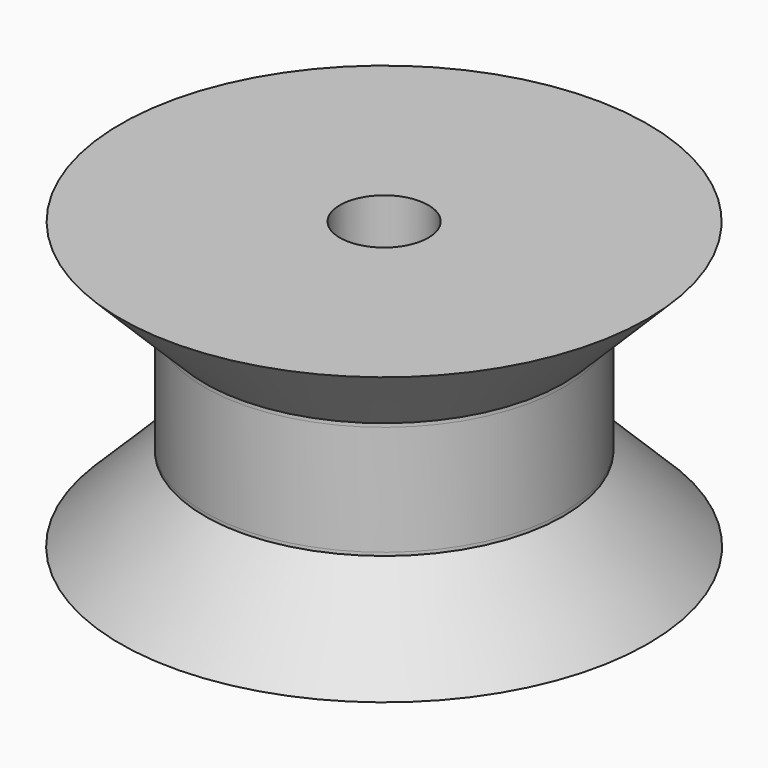
from build123d import *

# Parameters (mm, degrees)
F0_R        = 152.4
F1_DEPTH    = 50.8
F2_R        = 103.4812283395
F3_DEPTH    = 63.5
F5_R        = 152.1778472169
F6_DEPTH    = 50.8
F7_S5_R     = 103.4812283395
F7_T6_DEPTH = 218
F8_S5_R     = 103.4812283395
F8_T6_DEPTH = 219
F9_R        = 25.5370078958
F10_DEPTH   = 203.2


# Not quite as in the source:
# - a fillet or chamfer that OpenCascade refuses, or shapes differently, is made with other operations: its cross-section is extruded or revolved along the edge and cut away or added


with BuildPart() as f1:
    # F0 (on Top) → F1 (new body)
    with BuildSketch(Plane.XY):
        Circle(F0_R)
    extrude(amount=F1_DEPTH)

    # F2 (on face) → F3 (join)
    with BuildSketch(Plane.XY.offset(50.8)):
        Circle(F2_R)
    extrude(amount=F3_DEPTH)

    # F5 (on face) → F6 (join)
    with BuildSketch(Plane.XY.offset(114.3)):
        Circle(F5_R)
    extrude(amount=F6_DEPTH)

    # F7: chamfer of 50.8 on 1 edges, made by hand


with BuildPart() as f7_tool2:
    # F7_s3 → F7_t4 (revolve)
    with BuildSketch(Plane.XZ):
        Polygon((152.1778472169, 165.1), (101.3778472169, 114.3), (152.1778472169, 114.3), align=None)
    revolve(axis=Axis((0, 0, 114.3), (0, 0, 1)))

    # F7_s5 → F7_t6 (cut, symmetric)
    with BuildSketch(Plane.XY.offset(139.7)):
        Circle(F7_S5_R)
    extrude(amount=F7_T6_DEPTH, both=True, mode=Mode.SUBTRACT)


with BuildPart() as f1_1:
    add(f1.part)

    # F7_t1: cut F7_tool2
    add(f7_tool2.part, mode=Mode.SUBTRACT)

    # F8: chamfer of 50.8 on 1 edges, made by hand


with BuildPart() as f8_tool2:
    # F8_s3 → F8_t4 (revolve)
    with BuildSketch(Plane.XZ):
        Polygon((101.6, 50.8), (152.4, 0), (152.4, 50.8), align=None)
    revolve(axis=Axis((0, 0, 50.8), (0, 0, 1)))

    # F8_s5 → F8_t6 (cut, symmetric)
    with BuildSketch(Plane.XY.offset(25.4)):
        Circle(F8_S5_R)
    extrude(amount=F8_T6_DEPTH, both=True, mode=Mode.SUBTRACT)


with BuildPart() as f1_2:
    add(f1_1.part)

    # F8_t1: cut F8_tool2
    add(f8_tool2.part, mode=Mode.SUBTRACT)

    # F9 (on face) → F10 (cut)
    with BuildSketch(Plane.XY.offset(165.1)):
        Circle(F9_R)
    extrude(amount=-F10_DEPTH, mode=Mode.SUBTRACT)


solid = f1_2.part
